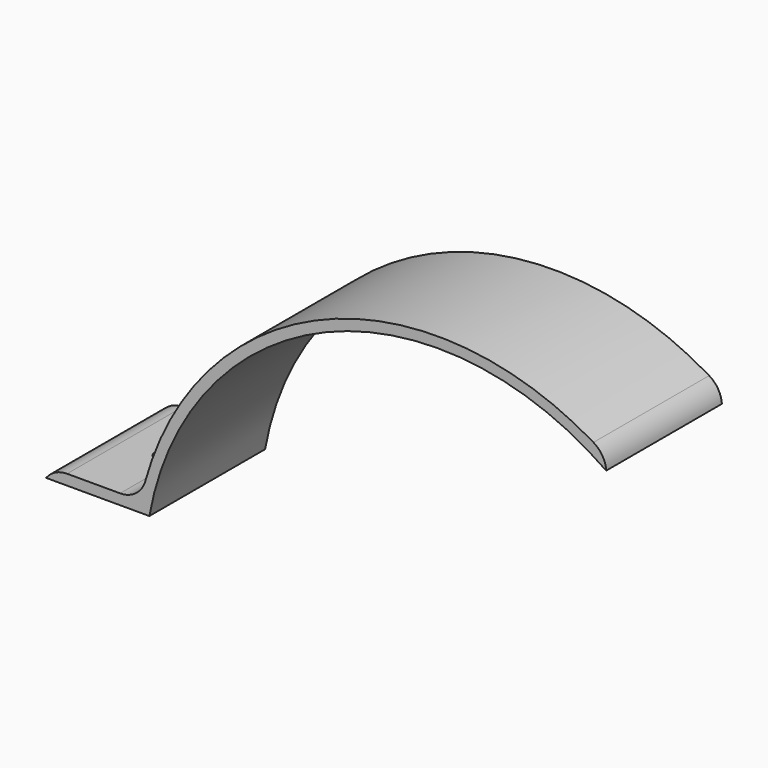
from build123d import *

# Parameters (mm, degrees)
F1_DEPTH    = 35
F2_T1_DEPTH = 35
F2_T3_DEPTH = 60.4
F2_T5_DEPTH = 62.0452734599
F3_R        = 2.5
F4_DEPTH    = 61.0006540296


# Not quite as in the source:
# - a fillet or chamfer that OpenCascade refuses, or shapes differently, is made with other operations: its cross-section is extruded or revolved along the edge and cut away or added


with BuildPart() as f1:
    # F0 (on Front) → F1 (new body)
    with BuildSketch(Plane.XZ):
        with BuildLine():
            Line((0, 2.54), (0, 0))
            Line((0, 0), (25, 0))
            ThreePointArc((25, 0), (67.7784437716, 53.0927080046), (135.550785483, 45.6267456604))
            Line((135.550785483, 45.6267456604), (137.0076696313, 47.7073918529))
            ThreePointArc((137.0076696313, 47.7073918529), (67.7975373338, 55.8400571127), (22.9055940849, 2.54))
            Line((22.9055940849, 2.54), (0, 2.54))
        make_face()
    extrude(amount=F1_DEPTH)

    # F2: fillet of radius 6.35 on 3 edges, made by hand

    # F2_s2 → F2_t1 (join)
    with BuildSketch(Plane.XZ):
        with BuildLine():
            ThreePointArc((17.9186335189, 2.54), (21.7605713102, 3.8341109577), (24.0365583001, 7.1889719661))
            ThreePointArc((24.0365583001, 7.1889719661), (23.4332372688, 4.8736911297), (22.9055940849, 2.54))
            Line((22.9055940849, 2.54), (17.9186335189, 2.54))
        make_face()
    extrude(amount=F2_T1_DEPTH)

    # F2_s4 → F2_t3 (cut)
    with BuildSketch(Plane.XZ.offset(-12.7)):
        with BuildLine():
            ThreePointArc((5.08, 2.54), (2.2401936686, 1.8696126628), (0, 0))
            Line((0, 0), (0, 2.54))
            Line((0, 2.54), (5.08, 2.54))
        make_face()
    extrude(amount=F2_T3_DEPTH, mode=Mode.SUBTRACT)

    # F2_s6 → F2_t5 (cut)
    with BuildSketch(Plane.XZ.offset(-13.52263673)):
        with BuildLine():
            ThreePointArc((132.4656708106, 50.6447579134), (134.6252880595, 48.5151252309), (135.550785483, 45.6267456604))
            Line((135.550785483, 45.6267456604), (137.0076696313, 47.7073918529))
            ThreePointArc((137.0076696313, 47.7073918529), (134.7637005445, 49.2178714094), (132.4656708106, 50.6447579134))
        make_face()
    extrude(amount=F2_T5_DEPTH, mode=Mode.SUBTRACT)

    # F3 (on face) → F4 (cut, through all)
    with BuildSketch(Plane(origin=(0, 0, 0), x_dir=(1, 0, 0), z_dir=(0, 0, -1))):
        with Locations((15, 17.5375)):
            Circle(F3_R)
    extrude(amount=-F4_DEPTH, mode=Mode.SUBTRACT)


solid = f1.part
